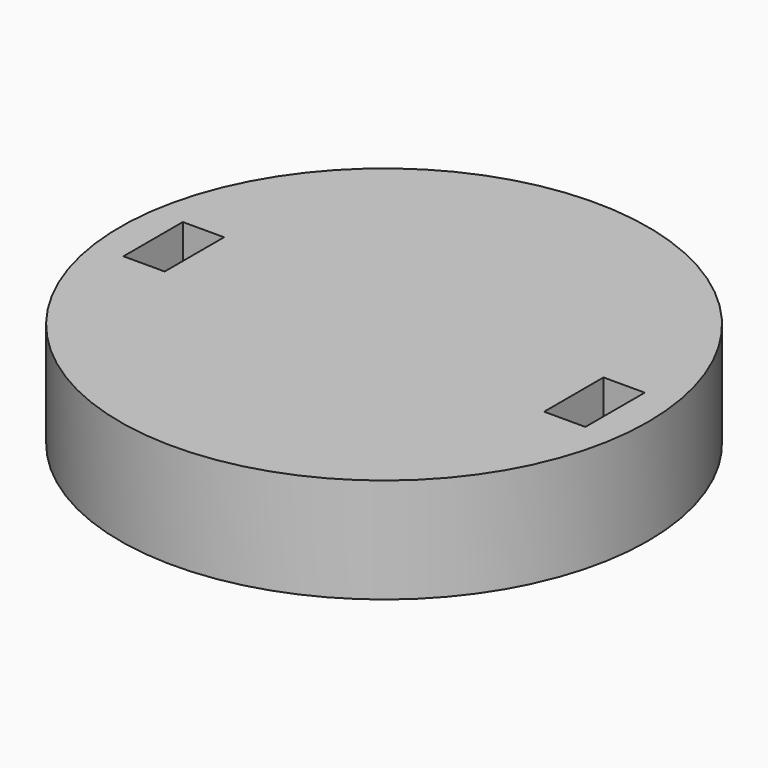
from build123d import *

# Parameters (mm, degrees)
F0_R     = 16
F0_W     = 2.5
F0_H     = 4.5
F1_DEPTH = 6.35


# Not quite as in the source:
# - a length typed as a fraction of an inch, garbled in the dataset ("3 / 203.2 mm" for 3/8 in), is restored


with BuildPart() as f1:
    # F0 (on Top) → F1 (new body)
    with BuildSketch(Plane.XY):
        Circle(F0_R)
        with Locations((-12.75, 0)):
            Rectangle(F0_W, F0_H, mode=Mode.SUBTRACT)
        with Locations((12.75, 0)):
            Rectangle(F0_W, F0_H, mode=Mode.SUBTRACT)
    extrude(amount=F1_DEPTH)


solid = f1.part
